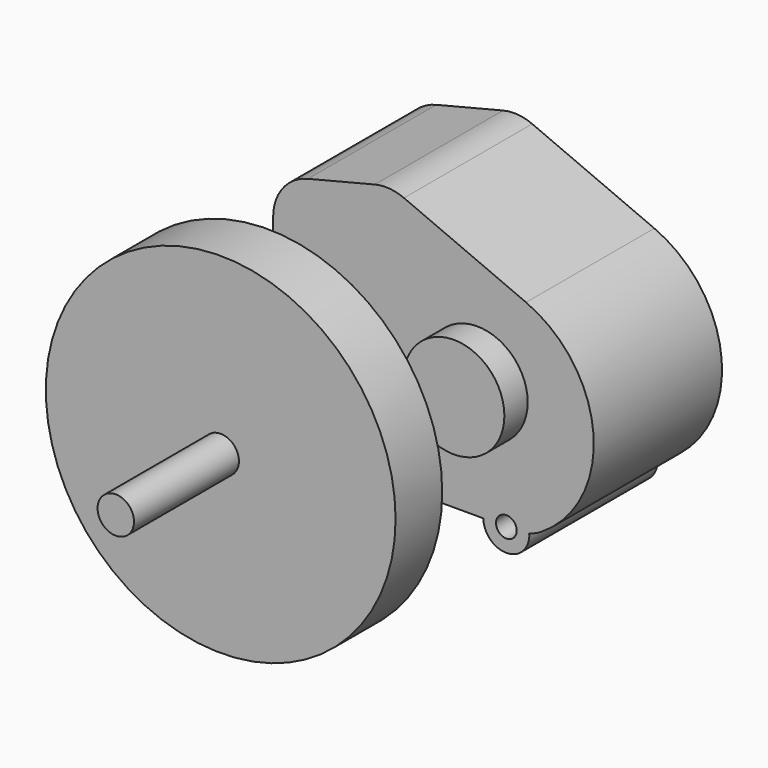
from build123d import *

# Parameters (mm, degrees)
F1_DEPTH      = 69.85
F2_R          = 22
F3_DEPTH      = 79.375
F3_DEPTH_BACK = 12.7
F4_R          = 10
F5_DEPTH      = 69.85
F6_R          = 4.5
F7_DEPTH      = 82.551
F8_R          = 19.05
F9_DEPTH      = 38.1
F10_R         = 7.9375
F11_DEPTH     = 82.55
F12_R         = 76.2
F13_DEPTH     = 25.4


# Not quite as in the source:
# - a length typed as a fraction of an inch, garbled in the dataset ("3 / 203.2 mm" for 3/8 in), is restored


with BuildPart() as f1:
    # F0 (on Front) → F1 (new body)
    with BuildSketch(Plane.XZ):
        with BuildLine():
            ThreePointArc((-32.4406404125, 46.3256966582), (-43.3540366721, 39.2310908433), (-47.5899279118, 26.9228466552))
            Line((-47.5899279118, 26.9228466552), (-47.5899279118, -33.6616252167))
            ThreePointArc((-47.5899279118, -33.6616252167), (-40.1504401539, -51.6221374588), (-22.1899279118, -59.0616252167))
            Line((-22.1899279118, -59.0616252167), (58.6284401518, -59.0616252167))
            ThreePointArc((58.6284401518, -59.0616252167), (64.1154300354, -58.2942262372), (69.1813488754, -56.0509194183))
            ThreePointArc((69.1813488754, -56.0509194183), (91.9687648373, -11.1091837062), (62.6034215093, 29.8383747833))
            Line((62.6034215093, 29.8383747833), (9.3969636816, 52.592505372))
            ThreePointArc((9.3969636816, 52.592505372), (3.1225085413, 54.1402430548), (-3.3179311218, 53.6063739808))
            Line((-3.3179311218, 53.6063739808), (-32.4406404125, 46.3256966582))
        make_face()
    extrude(amount=F1_DEPTH)

    # F2 (on face) → F3 (join, two sides)
    with BuildSketch(Plane.XZ.offset(69.85)) as f3_sk:
        with Locations((-9.4899279118, -20.9616252167)):
            Circle(F2_R)
        with Locations((41.3100720882, -8.2616252167)):
            Circle(F2_R)
    extrude(amount=-F3_DEPTH)
    extrude(f3_sk.sketch, amount=F3_DEPTH_BACK)

    # F4 (on face) → F5 (join, through all)
    with BuildSketch(Plane(origin=(0, 0, 0), x_dir=(-1, 0, 0), z_dir=(0, 1, 0))):
        with Locations((-54.0100720882, -59.0616252167)):
            Circle(F4_R)
        with Locations((3.1399279118, -59.0616252167)):
            Circle(F4_R)
    extrude(amount=-F5_DEPTH)

    # F6 (on face) → F7 (cut, through all)
    with BuildSketch(Plane(origin=(0, 0, 0), x_dir=(-1, 0, 0), z_dir=(0, 1, 0))):
        with Locations((-54.0100720882, -59.0616252167)):
            Circle(F6_R)
        with Locations((3.1399279118, -59.0616252167)):
            Circle(F6_R)
    extrude(amount=-F7_DEPTH, mode=Mode.SUBTRACT)

    # F8 (on face) → F9 (join)
    with BuildSketch(Plane.XZ.offset(82.55)):
        with Locations((-9.4899279118, -20.9616252167)):
            Circle(F8_R)
    extrude(amount=F9_DEPTH)

    # F10 (on face) → F11 (join)
    with BuildSketch(Plane.XZ.offset(120.65)):
        with Locations((-9.4899279118, -20.9616252167)):
            Circle(F10_R)
    extrude(amount=F11_DEPTH)

    # F12 (on face) → F13 (join)
    with BuildSketch(Plane.XZ.offset(120.65)):
        with Locations((-9.4899279118, -20.9616252167)):
            Circle(F12_R)
    extrude(amount=F13_DEPTH)


solid = f1.part
